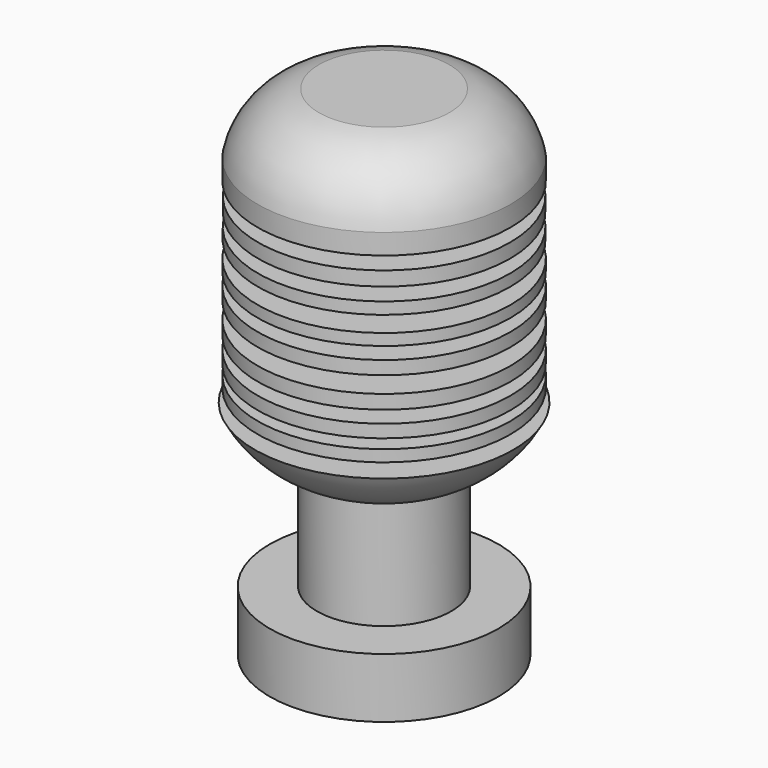
from build123d import *

# Parameters (mm, degrees)
F0_R     = 4
F1_DEPTH = 135


# Not quite as in the source:
# - a feature names something its author has since deleted; it is built from what else it names


with BuildPart() as f1:
    # F0 (on Top) → F1 (new body)
    with BuildSketch(Plane.XY):
        Circle(F0_R)
    extrude(amount=F1_DEPTH)


with BuildPart() as f3:
    # F2 (on Front) → F3 (revolve)
    with BuildSketch(Plane.XZ):
        with BuildLine():
            ThreePointArc((-5.4025318968, 144.3044847424), (-8.7187941889, 142.570608457), (-10.4812420468, 139.2694419797))
            Line((-10.4812420468, 139.2694419797), (-10.4812420468, 137.5795906956))
            Line((-10.4812420468, 137.5795906956), (-7.6773734327, 137.5795906956))
            Line((-7.6773734327, 137.5795906956), (-7.6773734327, 136.4770686801))
            Line((-7.6773734327, 136.4770686801), (-10.4469684447, 136.4770686801))
            Line((-10.4469684447, 136.4770686801), (-10.4469684447, 135.2973152099))
            Line((-10.4469684447, 135.2973152099), (-7.5175449747, 135.319129246))
            Line((-7.5175449747, 135.319129246), (-7.5175449747, 134.2156535561))
            Line((-7.5175449747, 134.2156535561), (-10.4518206354, 134.2156535561))
            Line((-10.4518206354, 134.2156535561), (-10.4518206354, 133.2342779811))
            Line((-10.4518206354, 133.2342779811), (-7.5175449747, 133.2342779811))
            Line((-7.5175449747, 133.2342779811), (-7.4386694032, 131.9274908478))
            Line((-7.4386694032, 131.9274908478), (-10.4812420468, 131.9274908478))
            Line((-10.4812420468, 131.9274908478), (-10.4812420468, 130.9773630078))
            Line((-10.4812420468, 130.9773630078), (-7.5752432022, 130.9773630078))
            Line((-7.5752432022, 130.9773630078), (-7.5752432022, 129.9533254082))
            Line((-7.5752432022, 129.9533254082), (-10.4812420468, 129.9533254082))
            Line((-10.4812420468, 129.9533254082), (-10.4812420468, 128.8439488585))
            Line((-10.4812420468, 128.8439488585), (-7.4899065803, 128.8439488585))
            Line((-7.4899065803, 128.8439488585), (-7.4899065803, 127.4785554583))
            Line((-7.4899065803, 127.4785554583), (-10.4812420468, 127.4785554583))
            Line((-10.4812420468, 127.4785554583), (-10.4812420468, 126.3265168841))
            Line((-10.4812420468, 126.3265168841), (-7.4899065803, 126.3265168841))
            Line((-7.4899065803, 126.3265168841), (-7.4899065803, 125.3024643834))
            Line((-7.4899065803, 125.3024643834), (-10.4812420468, 125.3024643834))
            Line((-10.4812420468, 125.3024643834), (-10.4812420468, 124.2357573087))
            Line((-10.4812420468, 124.2357573087), (-7.8191701323, 124.2357573087))
            Line((-7.8191701323, 124.2357573087), (-7.8191701323, 123.4466135502))
            Line((-7.8191701323, 123.4466135502), (-10.4812420468, 123.4466135502))
            Line((-10.4812420468, 123.4466135502), (-10.4812420468, 122.4818459327))
            Line((-10.4812420468, 122.4818459327), (-7.861838676, 122.4818459327))
            Line((-7.861838676, 122.4818459327), (-7.861838676, 121.4195713401))
            Line((-7.861838676, 121.4195713401), (-10.7123531493, 121.4195713401))
            ThreePointArc((-10.7123531493, 121.4195713401), (-8.6638063846, 118.8171942191), (-5.8128938955, 117.1316057444))
            Line((-5.8128938955, 117.1316057444), (-5.5729771993, 117.1316057444))
            Line((-5.5729771993, 117.1316057444), (-5.5729771993, 107.9735688748))
            Line((-5.5729771993, 107.9735688748), (-9.4849373709, 107.9735688748))
            Line((-9.4849373709, 107.9735688748), (-9.4849373709, 103.0133224906))
            Line((-9.4849373709, 103.0133224906), (0, 103.0133224906))
            Line((0, 103.0133224906), (0, 144.3145008144))
            Line((0, 144.3145008144), (-5.4025318968, 144.3044847424))
        make_face()
    revolve(axis=Axis((0, 0, 123.6639116525), (0, 0, 1)))

    # F4: cut F1
    add(f1.part, mode=Mode.SUBTRACT)


solid = f3.part
